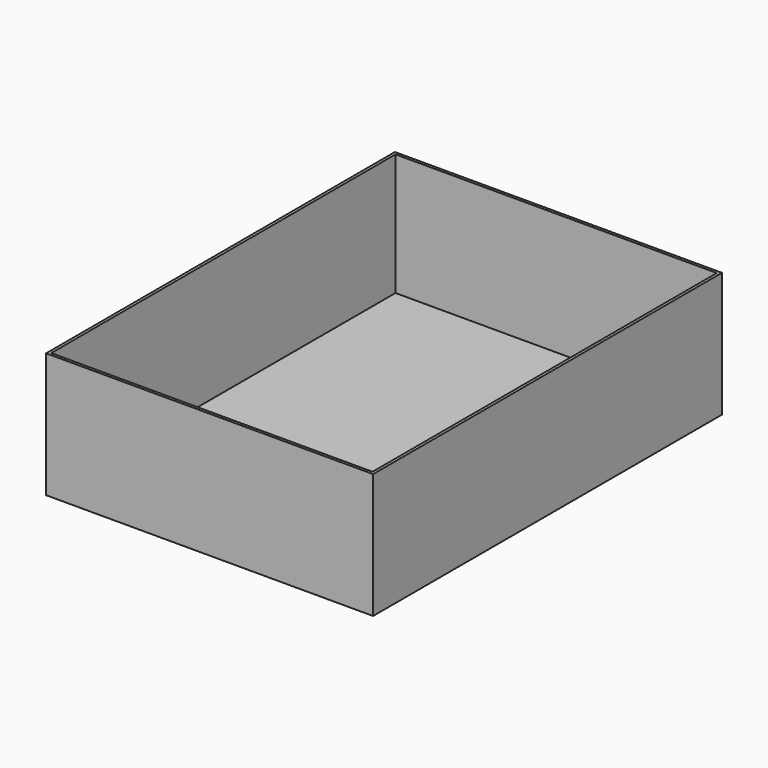
from build123d import *

# Parameters (mm, degrees)
F0_W     = 28.8
F0_H     = 38.4
F1_DEPTH = 11
F2_T     = -0.25


# Not quite as in the source:
# - the program builds the solid bodies; features that only make, move or delete a surface that nothing else refers to are left out


with BuildPart() as f1:
    # F0 (on Top) → F1 (new body)
    with BuildSketch(Plane.XY):
        with Locations((14.4, 19.2)):
            Rectangle(F0_W, F0_H)
    extrude(amount=F1_DEPTH)

    # F2
    f2_openings = [f1.faces().sort_by_distance(p)[0] for p in [
        (14.4, 19.2, 11),
    ]]
    offset(amount=F2_T, openings=f2_openings)


solid = f1.part
